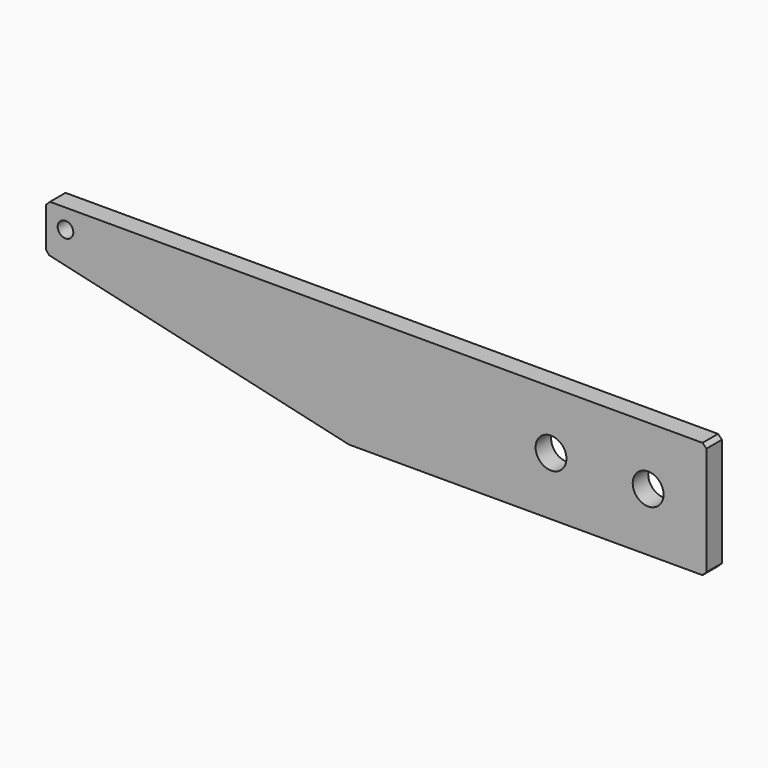
from build123d import *

# Parameters (mm, degrees)
F1_DEPTH    = 6.35
F2_T1_DEPTH = 12.8820747894
F2_T3_DEPTH = 11.6021811914
F4_D        = 10.0838
F6_D        = 5.1054


# Not quite as in the source:
# - a fillet or chamfer that OpenCascade refuses, or shapes differently, is made with other operations: its cross-section is extruded or revolved along the edge and cut away or added


with BuildPart() as f1:
    # F0 (on Front) → F1 (new body)
    with BuildSketch(Plane.XZ):
        Polygon((0, -38.1), (0, 0), (-215.9, 0), (-215.9, -15.24), (-116.8824615139, -38.1), align=None)
    extrude(amount=-F1_DEPTH)

    # F2: chamfer of 1.27 on 4 edges, made by hand

    # F2_s2 → F2_t1 (cut)
    with BuildSketch(Plane.XZ.offset(-9.6160373947)):
        Polygon((-214.63, 0), (-215.9, -1.27), (-215.9, 0), align=None)
        Polygon((-1.27, -38.1), (0, -36.83), (0, -38.1), align=None)
        Polygon((0, -1.27), (-1.27, 0), (0, 0), align=None)
    extrude(amount=F2_T1_DEPTH, mode=Mode.SUBTRACT)

    # F2_s4 → F2_t3 (cut)
    with BuildSketch(Plane.XZ.offset(-8.9760905957)):
        Polygon((-215.9, -14.2297963858), (-214.915687839, -15.4672463681), (-215.9, -15.24), align=None)
    extrude(amount=F2_T3_DEPTH, mode=Mode.SUBTRACT)

    # F4 (through all)
    with Locations(Plane.XZ):
        with Locations((-50.8, -19.05), (-19.05, -19.05)):
            Hole(F4_D / 2)

    # F6 (through all)
    with Locations(Plane.XZ):
        with Locations((-209.55, -6.35)):
            Hole(F6_D / 2)


solid = f1.part
